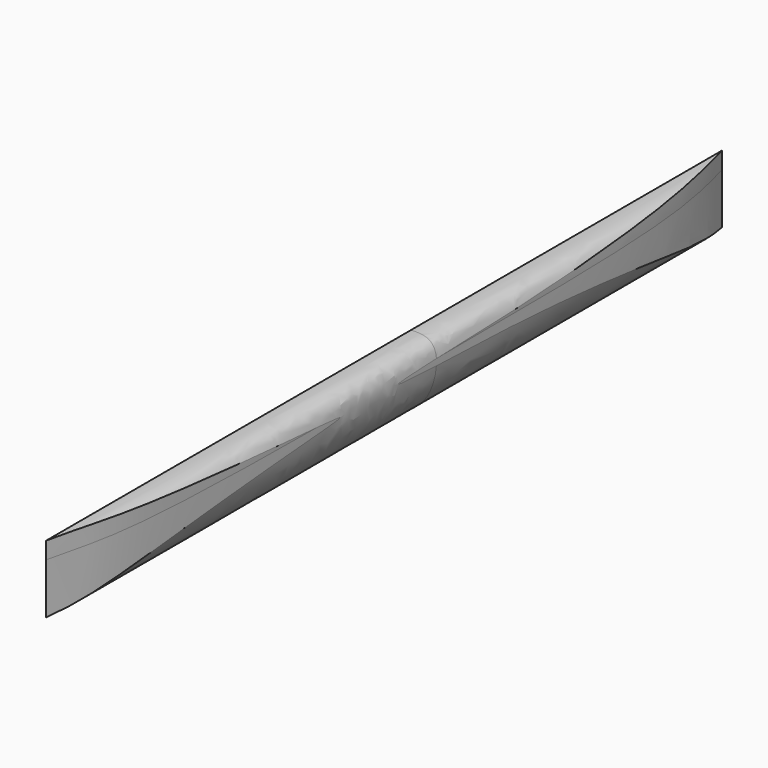
from build123d import *

# Parameters (mm, degrees)
F5_DEPTH = 5690
F6_DEPTH = 400


# Not quite as in the source:
# - the program builds the solid bodies; features that only make, move or delete a surface that nothing else refers to are left out


with BuildPart() as f5:
    # F2 (on Front) → F5 (new body, symmetric)
    with BuildSketch(Plane.XZ):
        with BuildLine():
            add(Edge.make_bspline(
                [(0, 100), (31.472475039, 101.2743608059), (104.0824556481, 102.4972249524), (184.410049505, 4.4962652473), (108.2069482323, -262.5694716116), (0, -300)],
                knots=[0, 0, 0, 0, 0.2548016815, 0.5225452679, 1, 1, 1, 1], degree=3))
            Line((0, 100), (0, -300))
        make_face()
    extrude(amount=F5_DEPTH, both=True)


with BuildPart() as f6:
    # F4 (on Top) → F6 (new body, symmetric)
    with BuildSketch(Plane.XY):
        with BuildLine():
            Line((0, 2300), (0, -2700))
            add(Edge.make_bspline(
                [(0, -2700), (33.1131047925, -2547.0221211395), (156.9449356141, -2173.0561860047), (149.0846675437, 15.3966573085), (146.8122429157, 1736.2105507374), (36.5493681578, 2169.0057550432), (0, 2300)],
                knots=[0, 0, 0, 0, 0.1678800286, 0.5166371664, 0.8321199714, 1, 1, 1, 1], degree=3))
        make_face()
    extrude(amount=F6_DEPTH, both=True)

    # F8: intersect F5
    add(f5.part, mode=Mode.INTERSECT)


solid = f6.part
